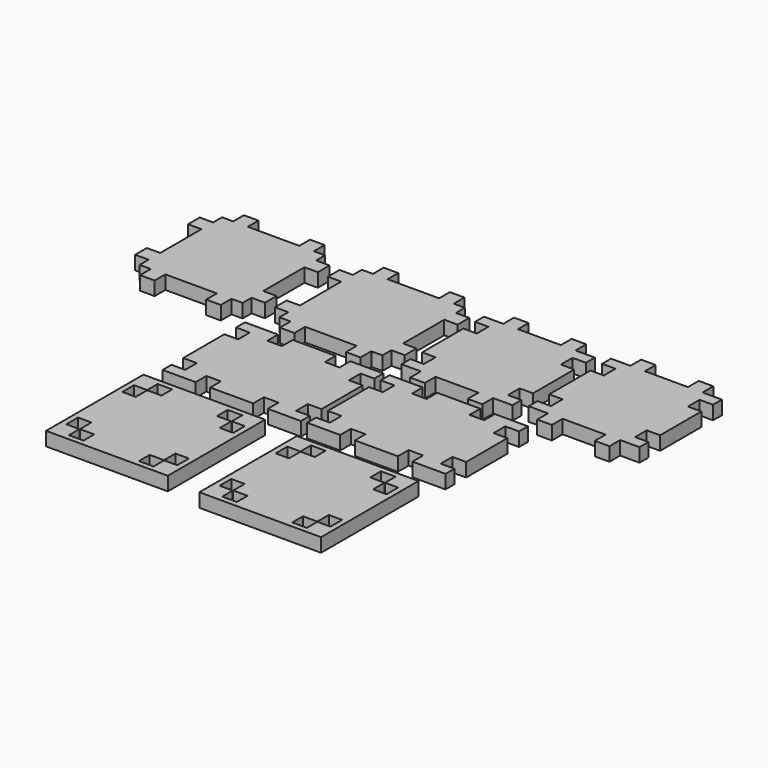
from build123d import *

# Parameters (mm, degrees)
F0_W     = 5.4
F0_H     = 4.953
F1_DEPTH = 5.08
F2_DEPTH = 5.07
F3_DEPTH = 5.08
F0_W_2   = 4.85
F0_H_2   = 4.85
F4_DEPTH = 5.08


# Not quite as in the source:
# - a feature names something its author has since deleted; it is built from what else it names


with BuildPart() as f1:
    # F0 (on Top) → F1 (new body)
    with BuildSketch(Plane.XY):
        Polygon((-40.8409686679, 41.5428522303), (-46.2409686087, 41.5429352911), (-46.2409686087, 41.5423593144), (-46.2417019953, 36.5893593687), (-40.8417020545, 36.5885597951), (-40.8409686679, 41.5415597408), align=None)
        Polygon((-16.3909687745, 41.5424761494), (-21.7909687745, 41.5425592102), (-21.7909687745, 41.5401493817), (-21.7909687745, 36.5871493817), (-16.3909687745, 36.5871493817), (-16.3909687745, 41.5401493817), align=None)
        Polygon((-12.2631478466, 51.0651565377), (-12.2631478466, 45.666827735), (-7.3129687762, 45.666827735), (-7.3129687762, 51.0650803959), align=None)
        Polygon((-12.2631478466, 75.5134995718), (-12.2631478466, 70.1151706882), (-7.3115584592, 70.1145136739), (-7.3107591443, 75.5127662756), align=None)
        Polygon((-55.3161478416, 70.1180676742), (-50.3631478421, 70.117991489), (-50.3631478421, 75.5163203351), (-55.3161478416, 75.5163203351), align=None)
        Polygon((-50.3653575284, 45.6696484078), (-50.3631478421, 45.6696484051), (-50.3631478421, 51.0679914933), (-50.3645582022, 51.0679771947), (-55.3175581586, 51.0686343962), (-55.3183574735, 45.6703817945), align=None)
        with Locations((-43.5381478433, 82.1194986883)):
            Rectangle(F0_W, F0_H)
        Polygon((-21.7874145632, 84.594588275), (-21.7881477411, 79.6429986883), (-16.3881476819, 79.6429986883), (-16.3874146224, 84.5937887014), align=None)
        Polygon((-50.3631478421, 45.6696484051), (-50.3631478421, 41.542998697), (-46.2409686087, 41.5429352911), (-40.8409686679, 41.5428522303), (-21.7909687745, 41.5425592102), (-16.3909687745, 41.5424761494), (-12.2631478466, 41.5424126568), (-12.2631478466, 45.666827735), (-12.2631478466, 51.0651565377), (-12.2631478466, 70.1151706882), (-12.2631478466, 75.5134995718), (-12.2631478466, 79.6429986883), (-16.3881476819, 79.6429986883), (-21.7881477411, 79.6429986883), (-31.3131478444, 79.6429986883), (-40.8381478433, 79.6429986883), (-46.2381478433, 79.6429986883), (-50.3631478421, 79.6429986883), (-50.3631478421, 75.5163203351), (-50.3631478421, 70.117991489), (-50.3631478421, 60.5929842896), (-50.3631478421, 51.0679914933), align=None)
    extrude(amount=F1_DEPTH)


with BuildPart() as f1b:
    # F0 (on Top) → F1, piece 2 (new body)
    with BuildSketch(Plane.XY):
        Polygon((-92.8586858753, 41.9452976998), (-98.2586858161, 41.9453807606), (-98.2586858161, 41.9448047839), (-98.2594192028, 36.9918048382), (-92.859419262, 36.9910052646), (-92.8586858753, 41.9440052103), align=None)
        Polygon((-68.408685982, 41.9449216189), (-73.808685982, 41.9450046798), (-73.808685982, 41.9425948512), (-73.808685982, 36.9895948512), (-68.408685982, 36.9895948512), (-68.408685982, 41.9425948512), align=None)
        Polygon((-64.2808650541, 51.4676020072), (-64.2808650541, 46.0692732045), (-59.3306859837, 46.0692732045), (-59.3306859837, 51.4675258654), align=None)
        Polygon((-64.2808650541, 75.9159450413), (-64.2808650541, 70.5176161577), (-59.3292756666, 70.5169591434), (-59.3284763517, 75.9152117451), align=None)
        Polygon((-107.333865049, 70.5205131437), (-102.3808650496, 70.5204369585), (-102.3808650496, 75.9187658046), (-107.333865049, 75.9187658046), align=None)
        Polygon((-102.3830747359, 46.0720938773), (-102.3808650496, 46.0720938747), (-102.3808650496, 51.4704369628), (-102.3822754097, 51.4704226642), (-107.3352753661, 51.4710798657), (-107.336074681, 46.072827264), align=None)
        with Locations((-95.5558650507, 82.5219441578)):
            Rectangle(F0_W, F0_H)
        Polygon((-73.8051317707, 84.9970337445), (-73.8058649486, 80.0454441578), (-68.4058648894, 80.0454441578), (-68.4051318299, 84.9962341709), align=None)
        Polygon((-102.3808650496, 46.0720938747), (-102.3808650496, 41.9454441665), (-98.2586858161, 41.9453807606), (-92.8586858753, 41.9452976998), (-73.808685982, 41.9450046798), (-68.408685982, 41.9449216189), (-64.2808650541, 41.9448581263), (-64.2808650541, 46.0692732045), (-64.2808650541, 51.4676020072), (-64.2808650541, 70.5176161577), (-64.2808650541, 75.9159450413), (-64.2808650541, 80.0454441578), (-68.4058648894, 80.0454441578), (-73.8058649486, 80.0454441578), (-83.3308650518, 80.0454441578), (-92.8558650507, 80.0454441578), (-98.2558650507, 80.0454441578), (-102.3808650496, 80.0454441578), (-102.3808650496, 75.9187658046), (-102.3808650496, 70.5204369585), (-102.3808650496, 60.9954297591), (-102.3808650496, 51.4704369628), align=None)
    extrude(amount=F1_DEPTH)


with BuildPart() as f1c:
    # F0 (on Top) → F1, piece 3 (new body)
    with BuildSketch(Plane.XY):
        with Locations((5.3587699927, 38.1856965442)):
            Rectangle(F0_W, F0_H)
        with Locations((26.6587699927, 38.1856965442)):
            Rectangle(F0_W, F0_H)
        with Locations((5.3587699927, 81.2386965442)):
            Rectangle(F0_W, F0_H)
        with Locations((26.6587699927, 81.2386965442)):
            Rectangle(F0_W, F0_H)
        Polygon((-4.4912300073, 44.7871965442), (-4.4912300073, 40.6621965442), (2.6587699927, 40.6621965442), (8.0587699927, 40.6621965442), (23.9587699927, 40.6621965442), (29.3587699927, 40.6621965442), (36.5087699927, 40.6621965442), (36.5087699927, 44.7871965442), (31.5557699927, 44.7871965442), (31.5557699927, 50.1871965442), (36.5087699927, 50.1871965442), (36.5087699927, 69.2371965442), (31.5557699927, 69.2371965442), (31.5557699927, 74.6371965442), (36.5087699927, 74.6371965442), (36.5087699927, 78.7621965442), (31.9087699927, 78.7621965442), (29.3587699927, 78.7621965442), (23.9587699927, 78.7621965442), (16.0087699927, 78.7621965442), (8.0587699927, 78.7621965442), (2.6587699927, 78.7621965442), (0.1087699927, 78.7621965442), (-4.4912300073, 78.7621965442), (-4.4912300073, 74.6371965442), (0.4617699927, 74.6371965442), (0.4617699927, 69.2371965442), (-4.4912300073, 69.2371965442), (-4.4912300073, 59.7121965442), (-4.4912300073, 50.1871965442), (0.4617699927, 50.1871965442), (0.4617699927, 44.7871965442), align=None)
    extrude(amount=F1_DEPTH)


with BuildPart() as f1d:
    # F0 (on Top) → F1, piece 4 (new body)
    with BuildSketch(Plane.XY):
        Polygon((-56.1625647761, -5.2273424947), (-51.0825647761, -5.2273424947), (-43.9325647761, -5.2273424947), (-43.9325647761, -0.2743424947), (-38.5325647761, -0.2743424947), (-38.5325647761, -5.2273424947), (-22.6325647761, -5.2273424947), (-22.6325647761, -0.2743424947), (-17.2325647761, -0.2743424947), (-17.2325647761, -5.2273424947), (-10.0825647761, -5.2273424947), (-5.0025647761, -5.2273424947), (-5.0025647761, -1.1023424947), (-10.0825647761, -1.1023424947), (-10.0825647761, 4.2976575053), (-5.0025647761, 4.2976575053), (-5.0025647761, 23.3476575053), (-10.0825647761, 23.3476575053), (-10.0825647761, 28.7476575053), (-5.0025647761, 28.7476575053), (-5.0025647761, 32.8726575053), (-10.0825647761, 32.8726575053), (-14.6825647761, 32.8726575053), (-17.2325647761, 32.8726575053), (-17.2325647761, 27.9196575053), (-22.6325647761, 27.9196575053), (-22.6325647761, 32.8726575053), (-30.5825647761, 32.8726575053), (-38.5325647761, 32.8726575053), (-38.5325647761, 27.9196575053), (-43.9325647761, 27.9196575053), (-43.9325647761, 32.8726575053), (-46.4825647761, 32.8726575053), (-51.0825647761, 32.8726575053), (-56.1625647761, 32.8726575053), (-56.1625647761, 28.7476575053), (-51.0825647761, 28.7476575053), (-51.0825647761, 23.3476575053), (-56.1625647761, 23.3476575053), (-56.1625647761, 4.2976575053), (-51.0825647761, 4.2976575053), (-51.0825647761, -1.1023424947), (-56.1625647761, -1.1023424947), align=None)
    extrude(amount=F1_DEPTH)


with BuildPart() as f2:
    # F0 (on Top) → F2 (new body)
    with BuildSketch(Plane.XY):
        Polygon((40.5567923505, 47.2221779553), (40.5567923505, 43.0971779553), (47.7067923505, 43.0971779553), (53.1067923505, 43.0971779553), (69.0067923505, 43.0971779553), (74.4067923505, 43.0971779553), (81.5567923505, 43.0971779553), (81.5567923505, 47.2221779553), (76.6037923505, 47.2221779553), (76.6037923505, 52.6221779553), (81.5567923505, 52.6221779553), (81.5567923505, 71.6721779553), (76.6037923505, 71.6721779553), (76.6037923505, 77.0721779553), (81.5567923505, 77.0721779553), (81.5567923505, 81.1971779553), (76.9567923505, 81.1971779553), (74.4067923505, 81.1971779553), (69.0067923505, 81.1971779553), (61.0567923505, 81.1971779553), (53.1067923505, 81.1971779553), (47.7067923505, 81.1971779553), (45.1567923505, 81.1971779553), (40.5567923505, 81.1971779553), (40.5567923505, 77.0721779553), (45.5097923505, 77.0721779553), (45.5097923505, 71.6721779553), (40.5567923505, 71.6721779553), (40.5567923505, 62.1471779553), (40.5567923505, 52.6221779553), (45.5097923505, 52.6221779553), (45.5097923505, 47.2221779553), align=None)
        with Locations((50.4067923505, 40.6206779553)):
            Rectangle(F0_W, F0_H)
        with Locations((71.7067923505, 40.6206779553)):
            Rectangle(F0_W, F0_H)
        with Locations((71.7067923505, 83.6736779553)):
            Rectangle(F0_W, F0_H)
        with Locations((50.4067923505, 83.6736779553)):
            Rectangle(F0_W, F0_H)
    extrude(amount=F2_DEPTH)


with BuildPart() as f3:
    # F0 (on Top) → F3 (new body)
    with BuildSketch(Plane.XY):
        Polygon((-2.9107588343, -4.9381693825), (2.1692411657, -4.9381693825), (9.3192411657, -4.9381693825), (9.3192411657, 0.0148306175), (14.7192411657, 0.0148306175), (14.7192411657, -4.9381693825), (30.6192411657, -4.9381693825), (30.6192411657, 0.0148306175), (36.0192411657, 0.0148306175), (36.0192411657, -4.9381693825), (43.1692411657, -4.9381693825), (48.2492411657, -4.9381693825), (48.2492411657, -0.8131693825), (43.1692411657, -0.8131693825), (43.1692411657, 4.5868306175), (48.2492411657, 4.5868306175), (48.2492411657, 23.6368306175), (43.1692411657, 23.6368306175), (43.1692411657, 29.0368306175), (48.2492411657, 29.0368306175), (48.2492411657, 33.1618306175), (43.1692411657, 33.1618306175), (38.5692411657, 33.1618306175), (36.0192411657, 33.1618306175), (36.0192411657, 28.2088306175), (30.6192411657, 28.2088306175), (30.6192411657, 33.1618306175), (22.6692411657, 33.1618306175), (14.7192411657, 33.1618306175), (14.7192411657, 28.2088306175), (9.3192411657, 28.2088306175), (9.3192411657, 33.1618306175), (6.7692411657, 33.1618306175), (2.1692411657, 33.1618306175), (-2.9107588343, 33.1618306175), (-2.9107588343, 29.0368306175), (2.1692411657, 29.0368306175), (2.1692411657, 23.6368306175), (-2.9107588343, 23.6368306175), (-2.9107588343, 4.5868306175), (2.1692411657, 4.5868306175), (2.1692411657, -0.8131693825), (-2.9107588343, -0.8131693825), align=None)
    extrude(amount=F3_DEPTH)


with BuildPart() as f3b:
    # F0 (on Top) → F3, piece 2 (new body)
    with BuildSketch(Plane.XY):
        Polygon((-36.1285774112, -12.9841668531), (-46.3785774112, -12.9841668531), (-46.3785774112, -17.9371668531), (-51.6755774112, -17.9371668531), (-51.6755774112, -23.2341668531), (-56.6285774112, -23.2341668531), (-56.6285774112, -43.7341668531), (-51.6755774112, -43.7341668531), (-51.6755774112, -49.0311668531), (-46.3785774112, -49.0311668531), (-46.3785774112, -53.9841668531), (-25.8785774112, -53.9841668531), (-25.8785774112, -49.0311668531), (-20.5815774112, -49.0311668531), (-20.5815774112, -43.7341668531), (-15.6285774112, -43.7341668531), (-15.6285774112, -33.4841668531), (-15.6285774112, -23.2341668531), (-20.5815774112, -23.2341668531), (-20.5815774112, -17.9371668531), (-25.8785774112, -17.9371668531), (-25.8785774112, -12.9841668531), align=None)
        with Locations((-54.2035774112, -15.4091668531)):
            Rectangle(F0_W_2, F0_H_2)
        with Locations((-54.2035774112, -51.5591668531)):
            Rectangle(F0_W_2, F0_H_2)
        Polygon((-56.6285774112, -17.8341668531), (-56.6285774112, -12.9841668531), (-56.6285774112, -10.9841668531), (-58.6285774112, -10.9841668531), (-58.6285774112, -53.9841668531), (-56.6285774112, -53.9841668531), (-56.6285774112, -49.1341668531), (-56.6285774112, -43.7341668531), (-56.6285774112, -23.2341668531), align=None)
        Polygon((-56.6285774112, -53.9841668531), (-58.6285774112, -53.9841668531), (-58.6285774112, -55.9841668531), (-13.6285774112, -55.9841668531), (-13.6285774112, -53.9841668531), (-15.6285774112, -53.9841668531), (-20.4785774112, -53.9841668531), (-25.8785774112, -53.9841668531), (-46.3785774112, -53.9841668531), (-51.7785774112, -53.9841668531), align=None)
        with Locations((-18.0535774112, -51.5591668531)):
            Rectangle(F0_W_2, F0_H_2)
        with Locations((-18.0535774112, -15.4091668531)):
            Rectangle(F0_W_2, F0_H_2)
        Polygon((-13.6285774112, -10.9841668531), (-15.6285774112, -10.9841668531), (-15.6285774112, -12.9841668531), (-15.6285774112, -17.8341668531), (-15.6285774112, -23.2341668531), (-15.6285774112, -33.4841668531), (-15.6285774112, -43.7341668531), (-15.6285774112, -49.1341668531), (-15.6285774112, -53.9841668531), (-13.6285774112, -53.9841668531), align=None)
        Polygon((-56.6285774112, -10.9841668531), (-56.6285774112, -12.9841668531), (-51.7785774112, -12.9841668531), (-46.3785774112, -12.9841668531), (-36.1285774112, -12.9841668531), (-25.8785774112, -12.9841668531), (-20.4785774112, -12.9841668531), (-15.6285774112, -12.9841668531), (-15.6285774112, -10.9841668531), align=None)
    extrude(amount=F3_DEPTH)


with BuildPart() as f4:
    # F0 (on Top) → F4 (new body)
    with BuildSketch(Plane.XY):
        Polygon((22.4280951531, -15.3173839013), (12.1780951531, -15.3173839013), (12.1780951531, -20.2703839013), (6.8810951531, -20.2703839013), (6.8810951531, -25.5673839013), (1.9280951531, -25.5673839013), (1.9280951531, -46.0673839013), (6.8810951531, -46.0673839013), (6.8810951531, -51.3643839013), (12.1780951531, -51.3643839013), (12.1780951531, -56.3173839013), (32.6780951531, -56.3173839013), (32.6780951531, -51.3643839013), (37.9750951531, -51.3643839013), (37.9750951531, -46.0673839013), (42.9280951531, -46.0673839013), (42.9280951531, -35.8173839013), (42.9280951531, -25.5673839013), (37.9750951531, -25.5673839013), (37.9750951531, -20.2703839013), (32.6780951531, -20.2703839013), (32.6780951531, -15.3173839013), align=None)
        Polygon((1.9280951531, -20.1673839013), (1.9280951531, -15.3173839013), (1.9280951531, -13.3173839013), (-0.0719048469, -13.3173839013), (-0.0719048469, -56.3173839013), (1.9280951531, -56.3173839013), (1.9280951531, -51.4673839013), (1.9280951531, -46.0673839013), (1.9280951531, -25.5673839013), align=None)
        with Locations((4.3530951531, -17.7423839013)):
            Rectangle(F0_W_2, F0_H_2)
        Polygon((1.9280951531, -13.3173839013), (1.9280951531, -15.3173839013), (6.7780951531, -15.3173839013), (12.1780951531, -15.3173839013), (22.4280951531, -15.3173839013), (32.6780951531, -15.3173839013), (38.0780951531, -15.3173839013), (42.9280951531, -15.3173839013), (42.9280951531, -13.3173839013), align=None)
        with Locations((40.5030951531, -17.7423839013)):
            Rectangle(F0_W_2, F0_H_2)
        Polygon((44.9280951531, -13.3173839013), (42.9280951531, -13.3173839013), (42.9280951531, -15.3173839013), (42.9280951531, -20.1673839013), (42.9280951531, -25.5673839013), (42.9280951531, -35.8173839013), (42.9280951531, -46.0673839013), (42.9280951531, -51.4673839013), (42.9280951531, -56.3173839013), (44.9280951531, -56.3173839013), align=None)
        with Locations((40.5030951531, -53.8923839013)):
            Rectangle(F0_W_2, F0_H_2)
        with Locations((4.3530951531, -53.8923839013)):
            Rectangle(F0_W_2, F0_H_2)
        Polygon((1.9280951531, -56.3173839013), (-0.0719048469, -56.3173839013), (-0.0719048469, -58.3173839013), (44.9280951531, -58.3173839013), (44.9280951531, -56.3173839013), (42.9280951531, -56.3173839013), (38.0780951531, -56.3173839013), (32.6780951531, -56.3173839013), (12.1780951531, -56.3173839013), (6.7780951531, -56.3173839013), align=None)
    extrude(amount=F4_DEPTH)


solid = Compound([f1.part, f1b.part, f1c.part, f1d.part, f2.part, f3.part, f3b.part, f4.part])
